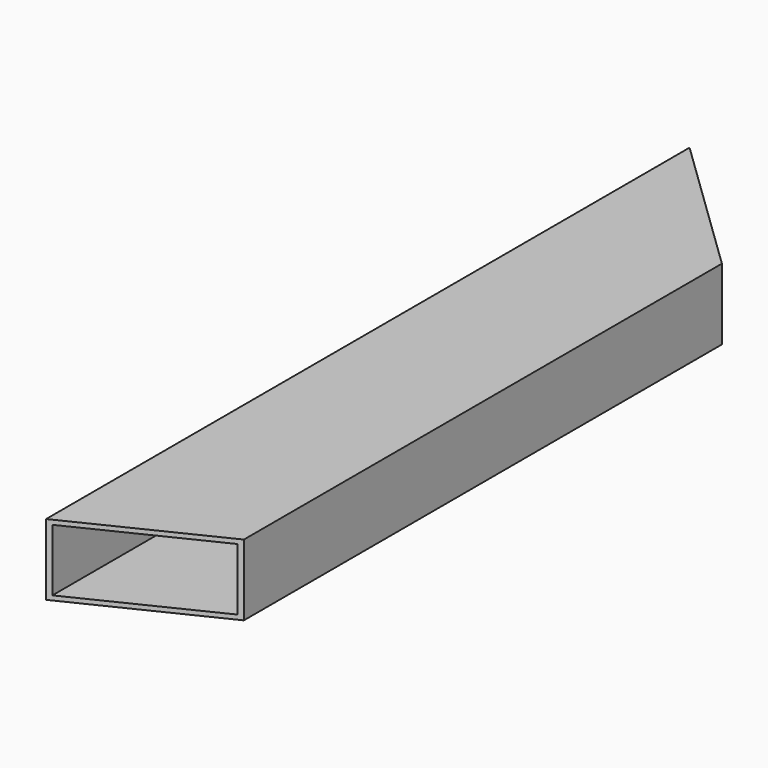
from build123d import *

# Parameters (mm, degrees)
F0_W        = 50
F0_H        = 25
F0_W_2      = 46.83
F0_H_2      = 21.83
F1_DEPTH    = 141.91
F2_T1_DEPTH = 288.1699043199
F3_T1_DEPTH = 286.404275023


# Not quite as in the source:
# - a fillet or chamfer that OpenCascade refuses, or shapes differently, is made with other operations: its cross-section is extruded or revolved along the edge and cut away or added


with BuildPart() as f1:
    # F0 (on Front) → F1 (new body, symmetric)
    with BuildSketch(Plane.XZ):
        Rectangle(F0_W, F0_H)
        Rectangle(F0_W_2, F0_H_2, mode=Mode.SUBTRACT)
    extrude(amount=F1_DEPTH, both=True)

    # F2: chamfer of 50.8 x 24.77 on 1 edges, made by hand

    # F2_s2 → F2_t1 (cut)
    with BuildSketch(Plane.XY.offset(-144.08495216)):
        Polygon((25, -117.14), (-25.8, -141.91), (25, -141.91), align=None)
    extrude(amount=F2_T1_DEPTH, mode=Mode.SUBTRACT)

    # F3: chamfer of 50.8 x 49.05 on 1 edges, made by hand

    # F3_s2 → F3_t1 (cut)
    with BuildSketch(Plane.XY.offset(-143.2021375115)):
        Polygon((-25.8, 141.91), (25, 92.86), (25, 141.91), align=None)
    extrude(amount=F3_T1_DEPTH, mode=Mode.SUBTRACT)


solid = f1.part
